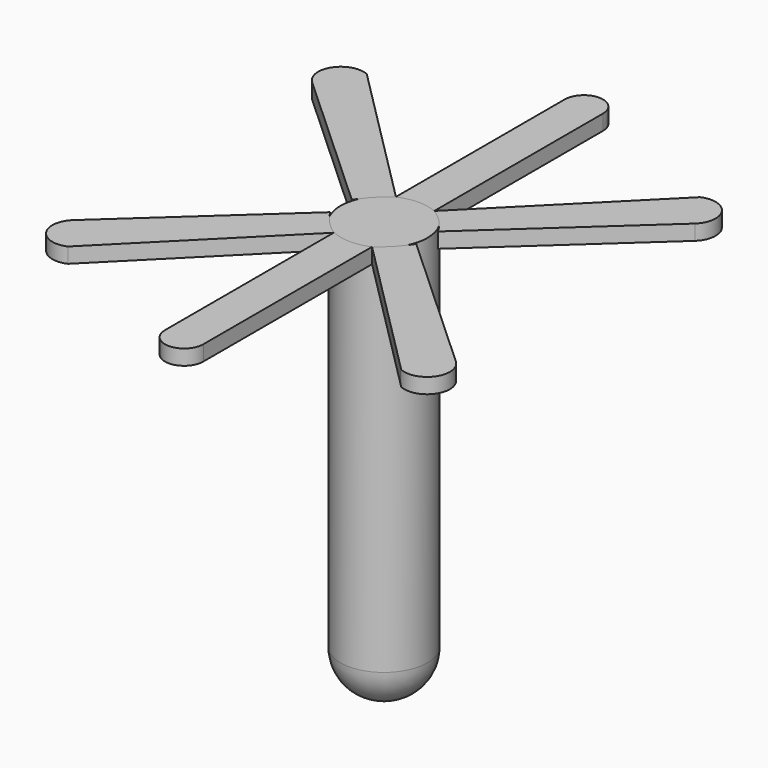
from build123d import *

# Parameters (mm, degrees)
F0_R     = 7.9646104271
F1_DEPTH = 76.2
F3_DEPTH = 1.27
F4_DEPTH = 2.794
F5_R     = 7.6651280605


with BuildPart() as f1:
    # F0 (on Top) → F1 (new body)
    with BuildSketch(Plane.XY):
        Circle(F0_R)
    extrude(amount=-F1_DEPTH)

    # F5
    f5_edges = [f1.edges().sort_by_distance(p)[0] for p in [
        (-7.96461, 0, -76.2),
    ]]
    fillet(f5_edges, radius=F5_R)


with BuildPart() as f3:
    # F2 (on Top) → F3 (new body)
    with BuildSketch(Plane.XY):
        with BuildLine():
            Line((-3.5088843636, 7.1228999505), (-3.5088843636, 7.0438587708))
            ThreePointArc((-3.5088843636, 7.0438587708), (-0.0085166469, 7.8395403691), (3.5088843636, 7.1228999505))
            Line((3.5088843636, 7.1228999505), (3.5088843636, 45.7731597126))
            ThreePointArc((3.5088843636, 45.7731597126), (0, 49.2820440761), (-3.5088843636, 45.7731597126))
            Line((-3.5088843636, 45.7731597126), (-3.5088843636, 7.1228999505))
        make_face()
    extrude(amount=-F3_DEPTH)

    # F2 (on Top) → F4, piece 3 (join)
    with BuildSketch(Plane.XY):
        with BuildLine():
            Line((-3.5088843636, 7.1228999505), (-3.5088843636, 7.0438587708))
            ThreePointArc((-3.5088843636, 7.0438587708), (-0.0085166469, 7.8395403691), (3.5088843636, 7.1228999505))
            Line((3.5088843636, 7.1228999505), (3.5088843636, 45.7731597126))
            ThreePointArc((3.5088843636, 45.7731597126), (0, 49.2820440761), (-3.5088843636, 45.7731597126))
            Line((-3.5088843636, 45.7731597126), (-3.5088843636, 7.1228999505))
        make_face()
    extrude(amount=-F4_DEPTH)


with BuildPart() as f4:
    # F2 (on Top) → F4 (new body)
    with BuildSketch(Plane.XY):
        with BuildLine():
            ThreePointArc((-7.8832879663, 2.4740586523), (-5.9135126334, 5.0030703093), (-3.5088843636, 7.1228999505))
            Line((-3.5088843636, 7.1228999505), (-30.534560875, 34.2191336145))
            ThreePointArc((-30.534560875, 34.2191336145), (-35.7195475655, 32.7132669375), (-35.0542927591, 27.3551742292))
            Line((-35.0542927591, 27.3551742292), (-7.8832879663, 2.4740586523))
        make_face()
    extrude(amount=-F4_DEPTH)


with BuildPart() as f4b:
    # F2 (on Top) → F4, piece 2 (new body)
    with BuildSketch(Plane.XY):
        with BuildLine():
            Line((30.534560875, 34.2191336145), (3.5088843636, 7.1228999505))
            ThreePointArc((3.5088843636, 7.1228999505), (6.0083363832, 5.0922962748), (7.8832879663, 2.4740586523))
            Line((7.8832879663, 2.4740586523), (35.0542927591, 27.3551742292))
            ThreePointArc((35.0542927591, 27.3551742292), (35.7195475655, 32.7132669375), (30.534560875, 34.2191336145))
        make_face()
    extrude(amount=-F4_DEPTH)


with BuildPart() as f4c:
    # F2 (on Top) → F4, piece 4 (new body)
    with BuildSketch(Plane.XY):
        with BuildLine():
            ThreePointArc((3.5088843636, -7.1228999505), (-0.0085166469, -7.8395403691), (-3.5088843636, -7.0438587708))
            Line((-3.5088843636, -7.0438587708), (-3.5088843636, -7.1228999505))
            Line((-3.5088843636, -7.1228999505), (-3.5088843636, -45.7731597126))
            ThreePointArc((-3.5088843636, -45.7731597126), (0, -49.2820440761), (3.5088843636, -45.7731597126))
            Line((3.5088843636, -45.7731597126), (3.5088843636, -7.1228999505))
        make_face()
    extrude(amount=-F4_DEPTH)


with BuildPart() as f4d:
    # F2 (on Top) → F4, piece 5 (new body)
    with BuildSketch(Plane.XY):
        with BuildLine():
            ThreePointArc((7.8832879663, -2.4740586523), (5.9191100309, -5.0083372725), (3.5088843636, -7.1228999505))
            Line((3.5088843636, -7.1228999505), (30.534560875, -34.2191336145))
            ThreePointArc((30.534560875, -34.2191336145), (35.7195475655, -32.7132669375), (35.0542927591, -27.3551742292))
            Line((35.0542927591, -27.3551742292), (7.8832879663, -2.4740586523))
        make_face()
    extrude(amount=-F4_DEPTH)


with BuildPart() as f4e:
    # F2 (on Top) → F4, piece 6 (new body)
    with BuildSketch(Plane.XY):
        with BuildLine():
            Line((-30.534560875, -34.2191336145), (-3.5088843636, -7.1228999505))
            ThreePointArc((-3.5088843636, -7.1228999505), (-5.9425805218, -5.0304222166), (-7.8832879663, -2.4740586523))
            Line((-7.8832879663, -2.4740586523), (-35.0542927591, -27.3551742292))
            ThreePointArc((-35.0542927591, -27.3551742292), (-35.7195475655, -32.7132669375), (-30.534560875, -34.2191336145))
        make_face()
    extrude(amount=-F4_DEPTH)


solid = Compound([f1.part, f3.part, f4.part, f4b.part, f4c.part, f4d.part, f4e.part])
